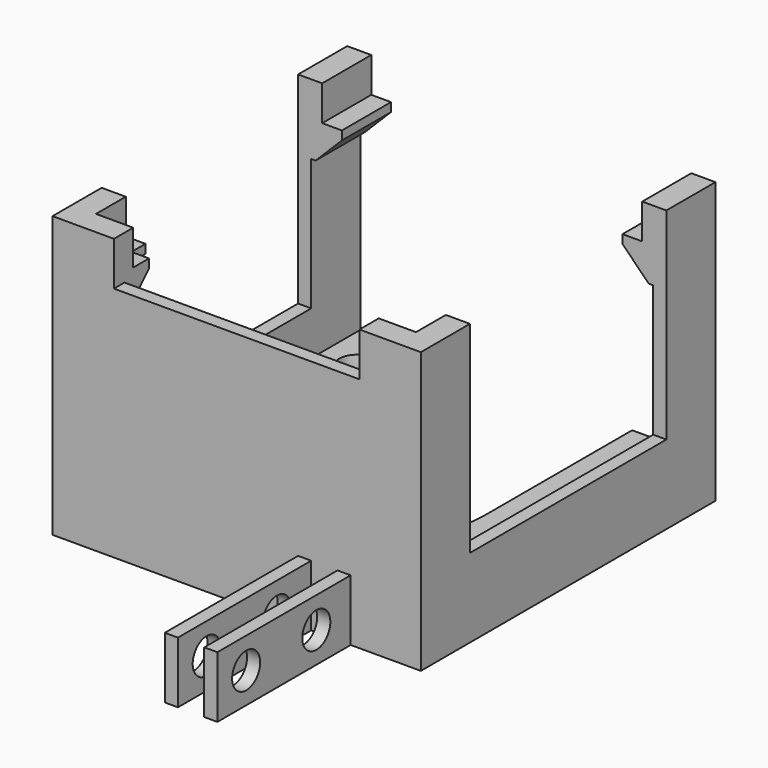
from build123d import *

# Parameters (mm, degrees)
F0_R      = 2
F0_W      = 1.5
F0_H      = 28
F0_W_2    = 28
F0_H_2    = 1.5
F0_W_3    = 8
F1_DEPTH  = 4
F2_DEPTH  = 23
F3_DEPTH  = 5
F4_W      = 2.75
F4_H      = 7
F5_DEPTH  = 5
F4_W_2    = 2.25
F6_DEPTH  = 1
F7_DEPTH  = 3
F8_SIZE   = 3
F9_W      = 1.5
F9_H      = 7
F10_DEPTH = 19
F11_R     = 2
F12_DEPTH = 14.001


# Not quite as in the source:
# - a feature names something its author has since deleted; it is built from what else it names


with BuildPart() as f1:
    # F0 (on Top) → F1 (new body)
    with BuildSketch(Plane.XY):
        with BuildLine():
            Line((-11.5, 19.5), (-19.5, 19.5))
            Line((-19.5, 19.5), (-19.5, 14))
            Line((-19.5, 14), (-19.5, -14))
            Line((-19.5, -14), (-19.5, -19.5))
            Line((-19.5, -19.5), (-14, -19.5))
            Line((-14, -19.5), (14, -19.5))
            Line((14, -19.5), (19.5, -19.5))
            Line((19.5, -19.5), (19.5, -14))
            Line((19.5, -14), (19.5, 14))
            Line((19.5, 14), (19.5, 19.5))
            Line((19.5, 19.5), (11.5, 19.5))
            Line((11.5, 19.5), (11.5, 0))
            ThreePointArc((11.5, 0), (0, -11.5), (-11.5, 0))
            Line((-11.5, 0), (-11.5, 19.5))
        make_face()
        with Locations((-15.5, -15.5)):
            Circle(F0_R, mode=Mode.SUBTRACT)
        with Locations((15.5, -15.5)):
            Circle(F0_R, mode=Mode.SUBTRACT)
        with Locations((-15.5, 15.5)):
            Circle(F0_R, mode=Mode.SUBTRACT)
        with Locations((15.5, 15.5)):
            Circle(F0_R, mode=Mode.SUBTRACT)
        with Locations((-20.25, 0)):
            Rectangle(F0_W, F0_H)
        Polygon((19.5, 21), (19.5, 19.5), (19.5, 14), (21, 14), (21, 21), align=None)
        Polygon((21, -14), (19.5, -14), (19.5, -19.5), (14, -19.5), (14, -21), (21, -21), align=None)
        Polygon((-19.5, -19.5), (-19.5, -14), (-21, -14), (-21, -21), (-14, -21), (-14, -19.5), align=None)
        Polygon((-19.5, 14), (-19.5, 19.5), (-19.5, 21), (-21, 21), (-21, 14), align=None)
        with Locations((20.25, 0)):
            Rectangle(F0_W, F0_H)
        with Locations((0, -20.25)):
            Rectangle(F0_W_2, F0_H_2)
        with Locations((-15.5, 20.25)):
            Rectangle(F0_W_3, F0_H_2)
        with Locations((15.5, 20.25)):
            Rectangle(F0_W_3, F0_H_2)
    extrude(amount=-F1_DEPTH)

    # F0 (on Top) → F2 (join)
    with BuildSketch(Plane.XY):
        Polygon((-19.5, -19.5), (-19.5, -14), (-21, -14), (-21, -21), (-14, -21), (-14, -19.5), align=None)
        Polygon((21, -14), (19.5, -14), (19.5, -19.5), (14, -19.5), (14, -21), (21, -21), align=None)
        Polygon((-19.5, 14), (-19.5, 19.5), (-19.5, 21), (-21, 21), (-21, 14), align=None)
        Polygon((19.5, 21), (19.5, 19.5), (19.5, 14), (21, 14), (21, 21), align=None)
        with Locations((0, -20.25)):
            Rectangle(F0_W_2, F0_H_2)
    extrude(amount=F2_DEPTH)

    # F0 (on Top) → F3 (join)
    with BuildSketch(Plane.XY):
        with Locations((20.25, 0)):
            Rectangle(F0_W, F0_H)
        with Locations((-20.25, 0)):
            Rectangle(F0_W, F0_H)
    extrude(amount=F3_DEPTH)

    # F4 (on face) → F5 (join)
    with BuildSketch(Plane.XY.offset(23)):
        with Locations((19.625, 17.5)):
            Rectangle(F4_W, F4_H)
        Polygon((14, -19.5), (14, -21), (21, -21), (21, -14), (19.5, -14), (19.5, -19.5), align=None)
        Polygon((-19.5, -19.5), (-21, -21), (-14, -21), (-14, -19.5), align=None)
        Polygon((-18.25, -18.25), (-19.5, -19.5), (-14, -19.5), (-14, -18.25), align=None)
        Polygon((-18.25, -14), (-19.5, -14), (-19.5, -19.5), (-18.25, -18.25), align=None)
        Polygon((-19.5, -14), (-21, -14), (-21, -21), (-19.5, -19.5), align=None)
        with Locations((-19.625, 17.5)):
            Rectangle(F4_W, F4_H)
        Polygon((14, -18.25), (14, -19.5), (19.5, -19.5), (19.5, -14), (18.25, -14), (18.25, -18.25), align=None)
    extrude(amount=F5_DEPTH)

    # F4 (on face) → F6 (join)
    with BuildSketch(Plane.XY.offset(23)):
        with Locations((17.125, 17.5)):
            Rectangle(F4_W_2, F4_H)
        Polygon((14, -16), (14, -18.25), (18.25, -18.25), (18.25, -14), (16, -14), (16, -16), align=None)
        Polygon((-16, -16), (-18.25, -18.25), (-14, -18.25), (-14, -16), align=None)
        Polygon((-16, -14), (-18.25, -14), (-18.25, -18.25), (-16, -16), align=None)
        with Locations((-17.125, 17.5)):
            Rectangle(F4_W_2, F4_H)
    extrude(amount=F6_DEPTH)

    # F7 (add): faces of the model
    f7_faces = [f1.faces().sort_by_distance(p)[0] for p in [
        (17.75, 17.5, 23),
        (17.0166666667, -17.0166666667, 23),
        (-17.0166666667, -17.0166666667, 23),
        (-17.75, 17.5, 23),
    ]]
    extrude(f7_faces, amount=F7_DEPTH)

    # F8
    f8_edges = [f1.edges().sort_by_distance(p)[0] for p in [
        (16, 17.5, 20),
        (15, -16, 20),
        (16, -15, 20),
        (-15, -16, 20),
        (-16, -15, 20),
        (-16, 17.5, 20),
    ]]
    chamfer(f8_edges, length=F8_SIZE)

    # F9 (on face) → F10 (join)
    with BuildSketch(Plane.XZ.offset(21)):
        with Locations((7.75, -0.5)):
            Rectangle(F9_W, F9_H)
        with Locations((12.25, -0.5)):
            Rectangle(F9_W, F9_H)
    extrude(amount=F10_DEPTH)

    # F11 (on face) → F12 (cut, through all)
    with BuildSketch(Plane(origin=(7, 0, 0), x_dir=(0, -1, 0), z_dir=(-1, 0, 0))):
        with Locations((25.9, -0.5)):
            Circle(F11_R)
        with Locations((35.9, -0.5)):
            Circle(F11_R)
    extrude(amount=-F12_DEPTH, mode=Mode.SUBTRACT)


solid = f1.part
